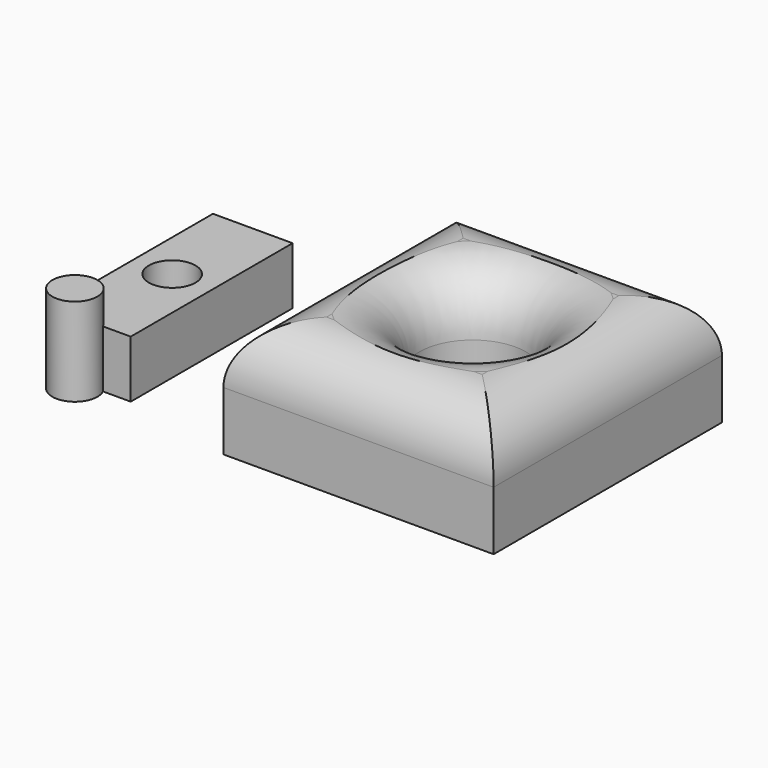
from build123d import *

# Parameters (mm, degrees)
F0_W        = 119.8333874345
F0_H        = 126.5625059605
F1_DEPTH    = 51.562
F2_R        = 23.5942925728
F3_DEPTH    = 115.824
F4_T1_DEPTH = 253.5625059605
F4_T3_DEPTH = 246.8333874345
F5_W        = 35.3249832988
F5_H        = 89.741922915
F5_R        = 10.343883472
F6_DEPTH    = 25.4
F7_R        = 9.9766133663
F8_DEPTH    = 39.116


# Not quite as in the source:
# - a fillet or chamfer that OpenCascade refuses, or shapes differently, is made with other operations: its cross-section is extruded or revolved along the edge and cut away or added


with BuildPart() as f1:
    # F0 (on Top) → F1 (new body)
    with BuildSketch(Plane.XY):
        Rectangle(F0_W, F0_H)
    extrude(amount=F1_DEPTH)

    # F2 (on face) → F3 (cut)
    with BuildSketch(Plane.XY.offset(51.562)):
        Circle(F2_R)
    extrude(amount=-F3_DEPTH, mode=Mode.SUBTRACT)

    # F4: fillet of radius 25.4 on 5 edges, made by hand

    # F4_s2 → F4_t1 (cut)
    with BuildSketch(Plane.XZ.offset(-126.7812529802)):
        with BuildLine():
            ThreePointArc((59.9166937172, 26.162), (52.4772059594, 44.1225122421), (34.5166937172, 51.562))
            Line((34.5166937172, 51.562), (59.9166937172, 51.562))
            Line((59.9166937172, 51.562), (59.9166937172, 26.162))
        make_face()
        with BuildLine():
            ThreePointArc((-34.5166937172, 51.562), (-52.4772059594, 44.1225122421), (-59.9166937172, 26.162))
            Line((-59.9166937172, 26.162), (-59.9166937172, 51.562))
            Line((-59.9166937172, 51.562), (-34.5166937172, 51.562))
        make_face()
    extrude(amount=F4_T1_DEPTH, mode=Mode.SUBTRACT)

    # F4_s4 → F4_t3 (cut)
    with BuildSketch(Plane.YZ.offset(-123.4166937172)):
        with BuildLine():
            ThreePointArc((-63.2812529802, 26.162), (-55.8417652224, 44.1225122421), (-37.8812529802, 51.562))
            Line((-37.8812529802, 51.562), (-63.2812529802, 51.562))
            Line((-63.2812529802, 51.562), (-63.2812529802, 26.162))
        make_face()
        with BuildLine():
            ThreePointArc((63.2812529802, 26.162), (55.8417652224, 44.1225122421), (37.8812529802, 51.562))
            Line((37.8812529802, 51.562), (63.2812529802, 51.562))
            Line((63.2812529802, 51.562), (63.2812529802, 26.162))
        make_face()
    extrude(amount=F4_T3_DEPTH, mode=Mode.SUBTRACT)

    # F4_s5 → F4_t6 (revolve, cut)
    with BuildSketch(Plane.XZ):
        with BuildLine():
            ThreePointArc((48.9942925728, 51.562), (31.0337803306, 44.1225122421), (23.5942925728, 26.162))
            Line((23.5942925728, 26.162), (23.5942925728, 51.562))
            Line((23.5942925728, 51.562), (48.9942925728, 51.562))
        make_face()
    revolve(axis=Axis((0, 0, 51.562), (0, 0, 1)), mode=Mode.SUBTRACT)


with BuildPart() as f6:
    # F5 (on Top) → F6 (new body)
    with BuildSketch(Plane.XY):
        with Locations((-127.3588873446, -7.5805075467)):
            Rectangle(F5_W, F5_H)
        with Locations((-127.7872473001, -6.8385624327)):
            Circle(F5_R, mode=Mode.SUBTRACT)
    extrude(amount=F6_DEPTH)

    # F7 (on Top) → F8 (join)
    with BuildSketch(Plane.XY):
        with Locations((-130.9662014246, -56.8105876446)):
            Circle(F7_R)
    extrude(amount=F8_DEPTH)


solid = Compound([f1.part, f6.part])
